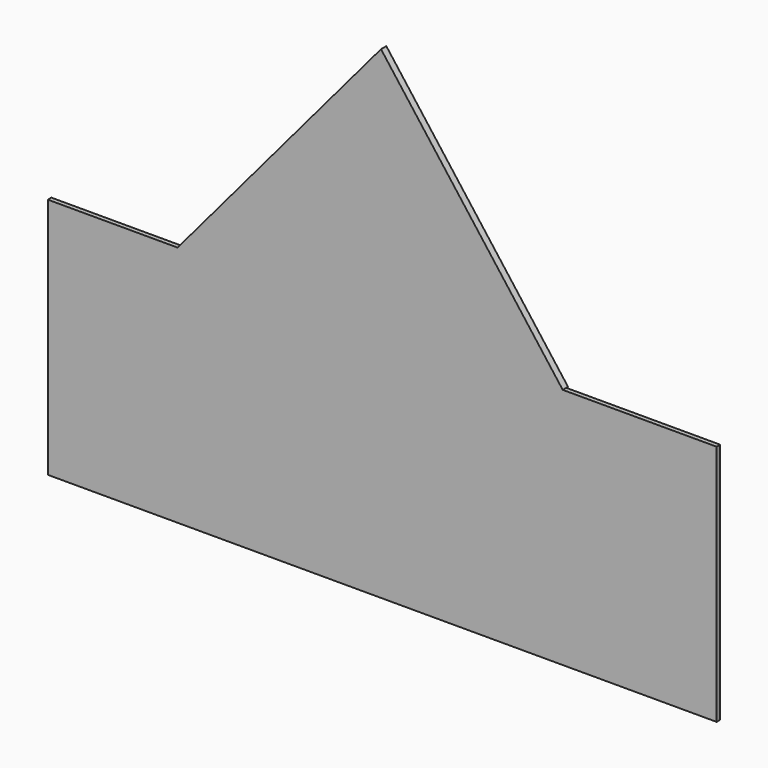
from build123d import *

# Parameters (mm, degrees)
F34_W     = 153.4406170249
F34_H     = 55.5722899735
F35_DEPTH = 0.762
F37_DEPTH = 1.27
F39_DEPTH = 0.254
F40_DEPTH = 0.254


# Not quite as in the source:
# - the program builds the solid bodies; features that only make, move or delete a surface that nothing else refers to are left out


with BuildPart() as f35:
    # F34 (on Front) → F35 (new body)
    with BuildSketch(Plane.XZ):
        with Locations((0.281136483, -27.7861449867)):
            Rectangle(F34_W, F34_H)
    extrude(amount=-F35_DEPTH)

    # F36 (on Front) → F37 (join)
    with BuildSketch(Plane.XZ):
        Polygon((41.6817590594, 0), (0, 55.2465841174), (-46.6600246727, 0), align=None)
    extrude(amount=-F37_DEPTH)

    # F38 (on face) → F39 (join)
    with BuildSketch(Plane(origin=(0, 1.27, 0), x_dir=(-1, 0, 0), z_dir=(0, 1, 0))):
        Polygon((46.6600246727, 0), (0, 55.2465841174), (-41.6817590594, 0), align=None)
    extrude(amount=F39_DEPTH)

    # F40 (add): a face of the model
    f40_faces = [f35.faces().sort_by_distance(p)[0] for p in [
        (0.281136483, 0.762, -27.7861449867),
    ]]
    extrude(f40_faces, amount=F40_DEPTH)


solid = f35.part
